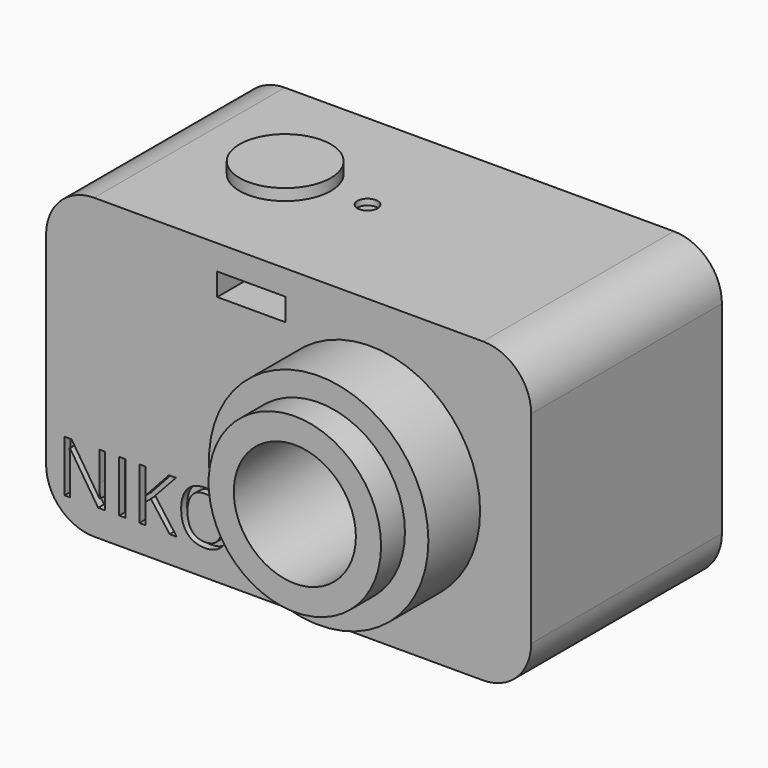
from build123d import *

# Parameters (mm, degrees)
F0_W          = 97.5468084216
F0_H          = 47.9522850364
F1_DEPTH      = 60
F2_R          = 9.6568542495
F3_R          = 22.0592859253
F4_DEPTH      = 13
F5_R          = 17.345185881
F6_DEPTH      = 6
F7_R          = 12.2780903553
F8_DEPTH      = 25
F9_R          = 9.1802336586
F10_DEPTH     = 2.3
F11_R         = 2.0330148181
F12_DEPTH     = 1.2
F13_W         = 13.7083334848
F13_H         = 4.5208334923
F14_DEPTH     = 69.5
F15_W         = 58.6046501994
F15_H         = 35.8953494579
F16_DEPTH     = 2.5
F17_T1_DEPTH  = 80.255285294
F17_T3_DEPTH  = 57.5459845525
F18_TEXT_SIZE = 14.5563920442
F19_DEPTH     = 1.5


# Not quite as in the source:
# - a fillet or chamfer that OpenCascade refuses, or shapes differently, is made with other operations: its cross-section is extruded or revolved along the edge and cut away or added
# - Text() gives the source's letters only with a copy of the font that has no kerning and outlines rounded to 1/6400 em; it was checked with that copy


with BuildPart() as f1:
    # F0 (on Top) → F1 (new body)
    with BuildSketch(Plane.XY):
        with Locations((-9.852103889, -0.9959200397)):
            Rectangle(F0_W, F0_H)
    extrude(amount=F1_DEPTH)

    # F2
    f2_edges = [f1.edges().sort_by_distance(p)[0] for p in [
        (38.9213, -0.99592, 60),
        (-58.625508, -0.99592, 60),
        (38.9213, -0.99592, 0),
        (-58.625508, -0.99592, 0),
    ]]
    fillet(f2_edges, radius=F2_R)

    # F3 (on face) → F4 (join)
    with BuildSketch(Plane.XZ.offset(24.9720625579)):
        with Locations((6.5973009914, 29.770469293)):
            Circle(F3_R)
    extrude(amount=F4_DEPTH)

    # F5 (on face) → F6 (join)
    with BuildSketch(Plane.XZ.offset(37.9720625579)):
        with Locations((6.5973009914, 29.770469293)):
            Circle(F5_R)
    extrude(amount=F6_DEPTH)

    # F7 (on face) → F8 (cut)
    with BuildSketch(Plane.XZ.offset(43.9720625579)):
        with Locations((6.5973009914, 29.770469293)):
            Circle(F7_R)
    extrude(amount=-F8_DEPTH, mode=Mode.SUBTRACT)

    # F9 (on face) → F10 (join)
    with BuildSketch(Plane.XY.offset(60)):
        with Locations((-30.5561702698, 0.0504448326)):
            Circle(F9_R)
    extrude(amount=F10_DEPTH)

    # F11 (on face) → F12 (cut)
    with BuildSketch(Plane.XY.offset(60)):
        with Locations((-13.9836696908, 0.0177775055)):
            Circle(F11_R)
    extrude(amount=-F12_DEPTH, mode=Mode.SUBTRACT)

    # F13 (on face) → F14 (cut)
    with BuildSketch(Plane(origin=(0, 22.9802224785, 0), x_dir=(-1, 0, 0), z_dir=(0, 1, 0))):
        with Locations((17.3541684635, 52.733335644)):
            Rectangle(F13_W, F13_H)
    extrude(amount=-F14_DEPTH, mode=Mode.SUBTRACT)

    # F15 (on face) → F16 (join)
    with BuildSketch(Plane(origin=(0, 22.9802224785, 0), x_dir=(-1, 0, 0), z_dir=(0, 1, 0))):
        with Locations((2.9302313924, 27.2124996409)):
            Rectangle(F15_W, F15_H)
    extrude(amount=F16_DEPTH)

    # F17: fillet of radius 5 on 4 edges, made by hand

    # F17_s2 → F17_t1 (cut)
    with BuildSketch(Plane.YZ.offset(-43.0578740394)):
        with BuildLine():
            ThreePointArc((22.9802224785, 45.1601743698), (24.8103494974, 43.3300473509), (25.4802224785, 40.8300473509))
            Line((25.4802224785, 40.8300473509), (25.4802224785, 45.1601743698))
            Line((25.4802224785, 45.1601743698), (22.9802224785, 45.1601743698))
        make_face()
        with BuildLine():
            ThreePointArc((22.9802224785, 9.264824912), (24.8103494974, 11.0949519309), (25.4802224785, 13.5949519309))
            Line((25.4802224785, 13.5949519309), (25.4802224785, 9.264824912))
            Line((25.4802224785, 9.264824912), (22.9802224785, 9.264824912))
        make_face()
    extrude(amount=F17_T1_DEPTH, mode=Mode.SUBTRACT)

    # F17_s4 → F17_t3 (cut)
    with BuildSketch(Plane.XY.offset(-1.5604926354)):
        with BuildLine():
            ThreePointArc((26.3720937073, 22.9802224785), (24.5419666884, 24.8103494974), (22.0419666884, 25.4802224785))
            Line((22.0419666884, 25.4802224785), (26.3720937073, 25.4802224785))
            Line((26.3720937073, 25.4802224785), (26.3720937073, 22.9802224785))
        make_face()
        with BuildLine():
            ThreePointArc((-32.2325564921, 22.9802224785), (-30.4024294732, 24.8103494974), (-27.9024294732, 25.4802224785))
            Line((-27.9024294732, 25.4802224785), (-32.2325564921, 25.4802224785))
            Line((-32.2325564921, 25.4802224785), (-32.2325564921, 22.9802224785))
        make_face()
    extrude(amount=F17_T3_DEPTH, mode=Mode.SUBTRACT)

    # F18 (on face) → F19 (cut)
    with BuildSketch(Plane.XZ.offset(24.9720625579)):
        with Locations((-56.3140422221, 5.3789485259)):
            Text('NIKON', F18_TEXT_SIZE, font='Open Sans', text_align=(TextAlign.LEFT, TextAlign.BOTTOM))
    extrude(amount=-F19_DEPTH, mode=Mode.SUBTRACT)


solid = f1.part
